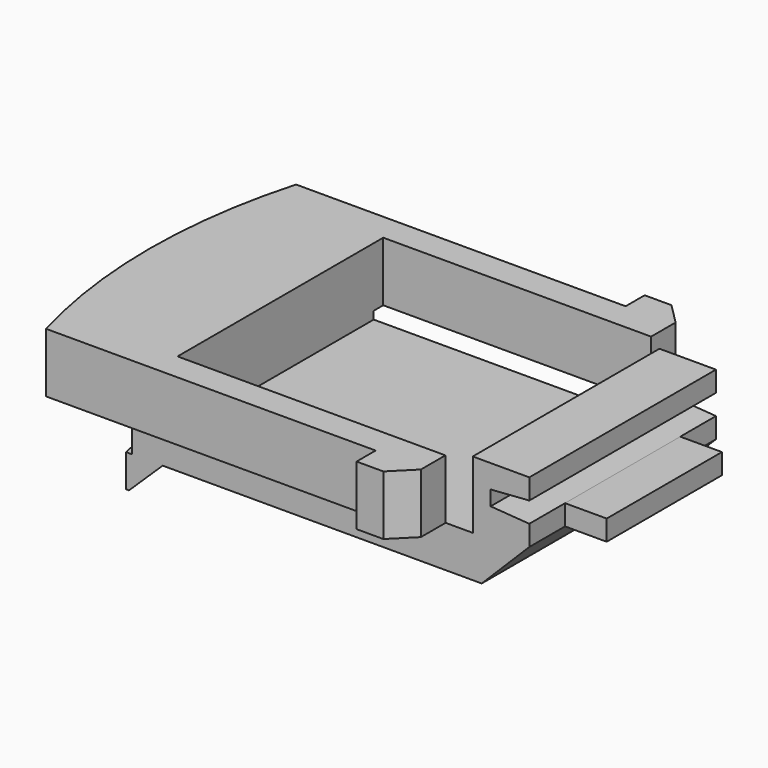
from build123d import *

# Parameters (mm, degrees)
F1_DEPTH  = 4.6482
F2_SIZE   = 2.032
F3_W      = 12.192
F3_H      = 2.8702
F4_DEPTH  = 4.9794
F6_DEPTH  = 1.397
F7_SIZE   = 1.39699
F9_DEPTH  = 4.9794
F10_W     = 3.0734
F10_H     = 0.8720666667
F11_DEPTH = 1.778
F13_DEPTH = 2.54
F14_SIZE  = 0.889


# Not quite as in the source:
# - a fillet or chamfer is up to 0.001 mm smaller than in the source, because OpenCascade refuses the exact size


with BuildPart() as f1:
    # F0 (on Top) → F1 (new body)
    with BuildSketch(Plane.XY):
        with BuildLine():
            Line((-21.8694, 0), (-4.3434, 0))
            Line((-4.3434, 0), (-4.3434, 4.9784))
            Line((-4.3434, 4.9784), (-21.2952151856, 4.9784))
            ThreePointArc((-21.2952151856, 4.9784), (-21.7253795748, 2.5057012372), (-21.8694, 0))
        make_face()
    extrude(amount=F1_DEPTH)

    # F2
    f2_edges = [f1.edges().sort_by_distance(p)[0] for p in [
        (-4.3434, 2.4892, 0),
    ]]
    chamfer(f2_edges, length=F2_SIZE)

    # F3 (on face) → F4 (cut, through all)
    with BuildSketch(Plane.XZ):
        with Locations((-12.8524, 3.2131)):
            Rectangle(F3_W, F3_H)
    extrude(amount=-F4_DEPTH, mode=Mode.SUBTRACT)

    # F5 (on face) → F6 (join)
    with BuildSketch(Plane(origin=(0, 0, 0), x_dir=(1, 0, 0), z_dir=(0, 0, -1))):
        with BuildLine():
            ThreePointArc((-22.1234, 0), (-21.9810877831, -2.5053158344), (-21.5559820236, -4.9784))
            Line((-21.5559820236, -4.9784), (-19.9887671906, -4.9784))
            ThreePointArc((-19.9887671906, -4.9784), (-20.4461719061, -2.5078546104), (-20.5994, 0))
            Line((-20.5994, 0), (-22.1234, 0))
        make_face()
    extrude(amount=F6_DEPTH)

    # F7 (size 1.397 in the source; OpenCascade refuses exactly that, so slightly less here)
    f7_edges = [f1.edges().sort_by_distance(p)[0] for p in [
        (-20.446172, 2.507855, -1.397),
    ]]
    chamfer(f7_edges, length=F7_SIZE)

    # F8 (on face) → F9 (cut, through all)
    with BuildSketch(Plane.XZ):
        Polygon((-4.3434, 2.9040666667), (-4.3434, 3.7761333333), (-5.9944, 3.6576), (-5.9944, 3.0226), align=None)
    extrude(amount=-F9_DEPTH, mode=Mode.SUBTRACT)

    # F10 (on face) → F11 (join)
    with BuildSketch(Plane.YZ.offset(-4.3434)):
        with Locations((1.5367, 2.4680333333)):
            Rectangle(F10_W, F10_H)
    extrude(amount=F11_DEPTH)

    # F12 (on face) → F13 (join)
    with BuildSketch(Plane.XY.offset(4.6482)):
        with BuildLine():
            Line((-24.5364, 0), (-18.9484, 0))
            Line((-18.9484, 0), (-18.9484, 5.4864))
            Line((-18.9484, 5.4864), (-7.5184, 5.4864))
            Line((-7.5184, 5.4864), (-7.5184, 7.6835))
            Line((-7.5184, 7.6835), (-9.5504, 7.6835))
            Line((-9.5504, 7.6835), (-9.5504, 6.6675))
            Line((-9.5504, 6.6675), (-23.6131185723, 6.6675))
            ThreePointArc((-23.6131185723, 6.6675), (-24.3044836141, 3.3655610544), (-24.5364, 0))
        make_face()
    extrude(amount=-F13_DEPTH)

    # F14
    f14_edges = [f1.edges().sort_by_distance(p)[0] for p in [
        (-7.5184, 7.6835, 3.3782),
    ]]
    chamfer(f14_edges, length=F14_SIZE)

    # F15: F1 across face


with BuildPart() as f1_1:
    add(f1.part)
    add(f1.part.mirror(Plane(origin=(-14.9823216408, 0, 1.8516826104), x_dir=(1, 0, 0), z_dir=(0, -1, 0))))


solid = f1_1.part
